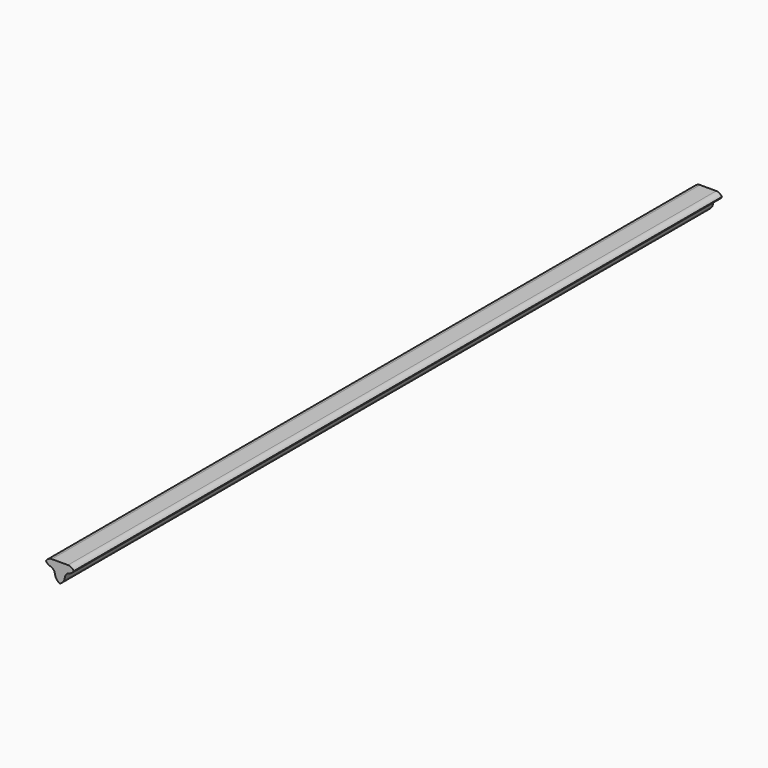
from build123d import *

# Parameters (mm, degrees)
F1_DEPTH    = 500.5
F2_R        = 4
F3_T1_DEPTH = 520.5
F3_T3_DEPTH = 519.2298334621
F4_T1_DEPTH = 525.22135955


# Not quite as in the source:
# - a fillet or chamfer that OpenCascade refuses, or shapes differently, is made with other operations: its cross-section is extruded or revolved along the edge and cut away or added


with BuildPart() as f1:
    # F0 (on Front) → F1 (new body)
    with BuildSketch(Plane.XZ):
        Polygon((9, 0), (0, 0), (-9, 0), (-9, -4), (-3, -4), (-3, -12), (3, -12), (3, -4), (9, -4), align=None)
    extrude(amount=F1_DEPTH)

    # F2
    f2_edges = [f1.edges().sort_by_distance(p)[0] for p in [
        (3, -250.25, -4),
        (-3, -250.25, -4),
    ]]
    fillet(f2_edges, radius=F2_R)

    # F3: fillet of radius 4 on 4 edges, made by hand

    # F3_s2 → F3_t1 (cut)
    with BuildSketch(Plane.XZ.offset(-10)):
        with BuildLine():
            ThreePointArc((-9, -4), (-7.8284271247, -1.1715728753), (-5, 0))
            Line((-5, 0), (-9, 0))
            Line((-9, 0), (-9, -4))
        make_face()
        with BuildLine():
            ThreePointArc((5, 0), (7.8284271247, -1.1715728753), (9, -4))
            Line((9, -4), (9, 0))
            Line((9, 0), (5, 0))
        make_face()
    extrude(amount=F3_T1_DEPTH, mode=Mode.SUBTRACT)

    # F3_s4 → F3_t3 (cut)
    with BuildSketch(Plane.XZ.offset(-9.364916731)):
        with BuildLine():
            ThreePointArc((-6, -4.1270166538), (-8.1622776602, -2.7035230504), (-9, -0.2540333076))
            Line((-9, -0.2540333076), (-9.4, -0.2540333076))
            Line((-9.4, -0.2540333076), (-9.4, -4))
            Line((-9.4, -4), (-9, -4.4))
            ThreePointArc((-9, -4.4), (-7, -4.4), (-6.1, -4.5143149884))
            Line((-6.1, -4.5143149884), (-6, -4.1270166538))
        make_face()
        with BuildLine():
            ThreePointArc((9, -0.2540333076), (8.1622776602, -2.7035230504), (6, -4.1270166538))
            Line((6, -4.1270166538), (6.1, -4.5143149884))
            ThreePointArc((6.1, -4.5143149884), (7, -4.4), (9, -4.4))
            Line((9, -4.4), (9.4, -4))
            Line((9.4, -4), (9.4, -0.2540333076))
            Line((9.4, -0.2540333076), (9, -0.2540333076))
        make_face()
    extrude(amount=F3_T3_DEPTH, mode=Mode.SUBTRACT)

    # F4: fillet of radius 5 on 2 edges, made by hand

    # F4_s2 → F4_t1 (cut)
    with BuildSketch(Plane.XZ.offset(-12.360679775)):
        with BuildLine():
            ThreePointArc((3.02476804, -7.5555555556), (1.3890614233, -10.7267799625), (-1.94427191, -12))
            Line((-1.94427191, -12), (-1.94427191, -12.5))
            Line((-1.94427191, -12.5), (3, -12.5))
            Line((3, -12.5), (3.5, -12))
            ThreePointArc((3.5, -12), (3.5, -8), (3.521672035, -7.6111111111))
            Line((3.521672035, -7.6111111111), (3.02476804, -7.5555555556))
        make_face()
        with BuildLine():
            ThreePointArc((1.94427191, -12), (-1.3890614233, -10.7267799625), (-3.02476804, -7.5555555556))
            Line((-3.02476804, -7.5555555556), (-3.521672035, -7.6111111111))
            ThreePointArc((-3.521672035, -7.6111111111), (-3.5, -8), (-3.5, -12))
            Line((-3.5, -12), (-3, -12.5))
            Line((-3, -12.5), (1.94427191, -12.5))
            Line((1.94427191, -12.5), (1.94427191, -12))
        make_face()
    extrude(amount=F4_T1_DEPTH, mode=Mode.SUBTRACT)


solid = f1.part
